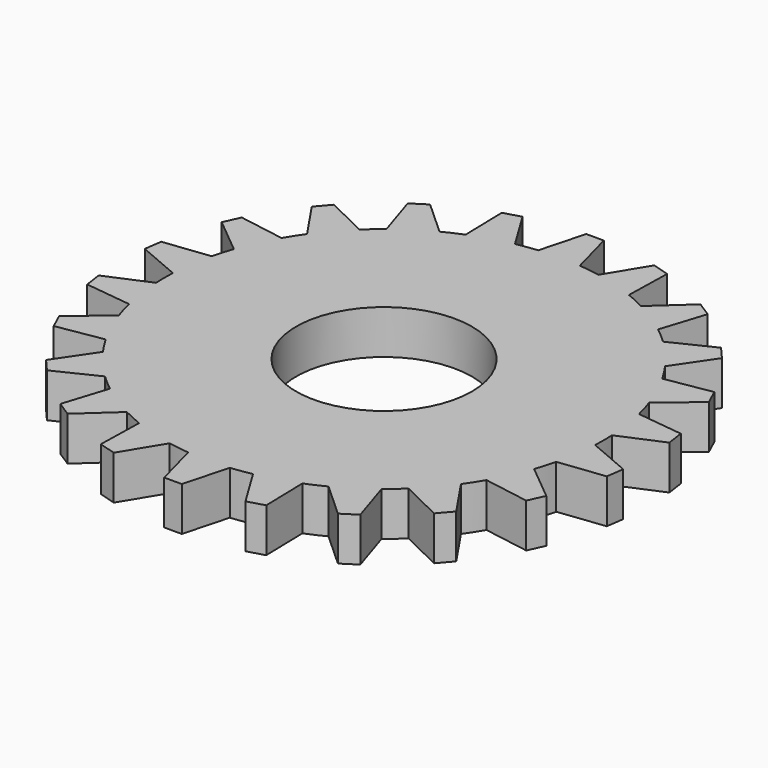
from build123d import *

# Parameters (mm, degrees)
F0_R            = 12.7
F0_R_2          = 5.08
F1_DEPTH        = 2.54
F3_DEPTH        = 2.54
F3_COPIES_COUNT = 22


# Not quite as in the source:
# - a pattern or mirror of a feature is missing from the dataset's text; its kind, count and spacing are read off the source's solid
# - a feature names something its author has since deleted; it is built from what else it names


with BuildPart() as f1:
    # F0 (on Top) → F1 (new body)
    with BuildSketch(Plane.XY):
        Circle(F0_R)
        Circle(F0_R_2, mode=Mode.SUBTRACT)
    extrude(amount=F1_DEPTH)

    # F2 (on face) → F3 (join)
    with BuildSketch(Plane.XY.offset(2.54)):
        with BuildLine():
            ThreePointArc((-1.2039155713, 12.64280773), (0, 12.7), (1.2039155713, 12.64280773))
            Line((1.2039155713, 12.64280773), (0.508, 15.24))
            Line((0.508, 15.24), (0, 15.24))
            Line((0, 15.24), (-0.508, 15.24))
            Line((-0.508, 15.24), (-1.2039155713, 12.64280773))
        make_face()
    f3 = extrude(amount=-F3_DEPTH)

    # F3_copies: F3 ×22 about axis
    f3_copies_axis = Axis((0, 0, 0), (0, 0, 1))
    for i in range(1, F3_COPIES_COUNT):
        add(f3.rotate(f3_copies_axis, i * 360 / F3_COPIES_COUNT))


solid = f1.part
